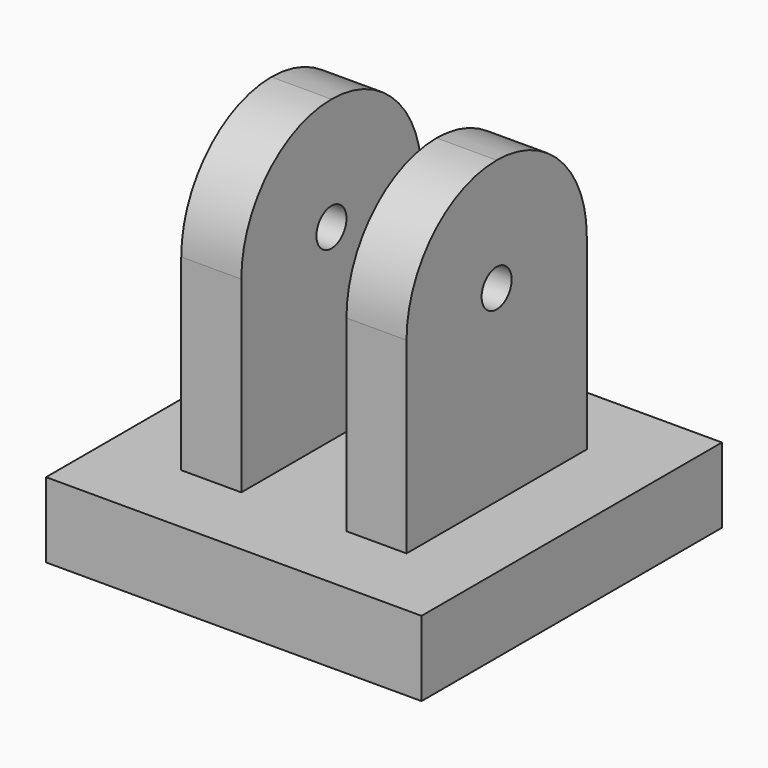
from build123d import *

# Parameters (mm, degrees)
F0_W     = 50
F0_H     = 50
F1_DEPTH = 10
F3_W     = 8
F3_H     = 30
F4_DEPTH = 40
F2_W     = 8
F2_H     = 30
F5_DEPTH = 40
F6_R     = 14.99999
F8_D     = 5


# Not quite as in the source:
# - a fillet or chamfer is up to 0.001 mm smaller than in the source, because OpenCascade refuses the exact size


with BuildPart() as f1:
    # F0 (on Top) → F1 (new body)
    with BuildSketch(Plane.XY):
        with Locations((-19.0450707451, -19.6881243537)):
            Rectangle(F0_W, F0_H)
    extrude(amount=F1_DEPTH)

    # F3 (on face) → F4 (join)
    with BuildSketch(Plane.XY.offset(10)):
        with Locations((-8.0450707451, -19.6881243537)):
            Rectangle(F3_W, F3_H)
    extrude(amount=F4_DEPTH)

    # F2 (on face) → F5 (join)
    with BuildSketch(Plane.XY.offset(10)):
        with Locations((-30.0450707451, -19.6881243537)):
            Rectangle(F2_W, F2_H)
    extrude(amount=F5_DEPTH)

    # F6 (radius 15 in the source; OpenCascade refuses exactly that, so slightly less here)
    f6_edges = [f1.edges().sort_by_distance(p)[0] for p in [
        (-8.045071, -4.688124, 50),
        (-30.045071, -4.688124, 50),
        (-8.045071, -34.688124, 50),
        (-30.045071, -34.688124, 50),
    ]]
    fillet(f6_edges, radius=F6_R)

    # F8 (through all)
    with Locations(Plane.YZ.offset(-4.0450707451)):
        with Locations((-19.6881243537, 35)):
            Hole(F8_D / 2)


solid = f1.part
